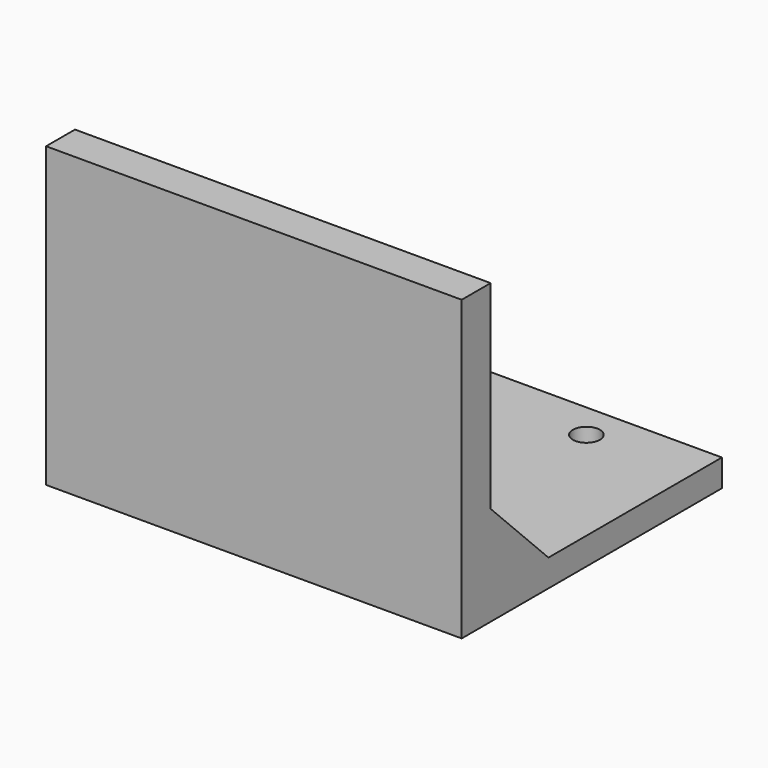
from build123d import *

# Parameters (mm, degrees)
F0_W      = 58.42
F0_H      = 45.72
F1_DEPTH  = 3.81
F2_W      = 58.42
F2_H      = 5.08
F3_DEPTH  = 38.1
F4_R      = 1.905
F5_DEPTH  = 3.811
F6_W      = 10.16
F6_H      = 10.16
F7_DEPTH  = 5.08
F8_SIZE   = 10.15999
F9_W      = 10.16
F9_H      = 10.16
F10_DEPTH = 5.08
F11_SIZE  = 10.15999


# Not quite as in the source:
# - a fillet or chamfer is up to 0.001 mm smaller than in the source, because OpenCascade refuses the exact size


with BuildPart() as f1:
    # F0 (on Top) → F1 (new body)
    with BuildSketch(Plane.XY):
        Rectangle(F0_W, F0_H)
    extrude(amount=F1_DEPTH)

    # F2 (on face) → F3 (join)
    with BuildSketch(Plane.XY.offset(3.81)):
        with Locations((0, -20.32)):
            Rectangle(F2_W, F2_H)
    extrude(amount=F3_DEPTH)

    # F4 (on face) → F5 (cut, through all)
    with BuildSketch(Plane.XY.offset(3.81)):
        with Locations((-14.224, 17.78)):
            Circle(F4_R)
        with Locations((14.224, 17.78)):
            Circle(F4_R)
        with Locations((14.224, -10.668)):
            Circle(F4_R)
        with Locations((-14.224, -10.668)):
            Circle(F4_R)
    extrude(amount=-F5_DEPTH, mode=Mode.SUBTRACT)

    # F6 (on face) → F7 (join)
    with BuildSketch(Plane(origin=(-29.21, 0, 0), x_dir=(0, -1, 0), z_dir=(-1, 0, 0))):
        with Locations((12.7, 8.89)):
            Rectangle(F6_W, F6_H)
    extrude(amount=-F7_DEPTH)

    # F8 (size 10.16 in the source; OpenCascade refuses exactly that, so slightly less here)
    f8_edges = [f1.edges().sort_by_distance(p)[0] for p in [
        (-26.67, -7.62, 13.97),
    ]]
    chamfer(f8_edges, length=F8_SIZE)

    # F9 (on face) → F10 (join)
    with BuildSketch(Plane.YZ.offset(29.21)):
        with Locations((-12.7, 8.89)):
            Rectangle(F9_W, F9_H)
    extrude(amount=-F10_DEPTH)

    # F11 (size 10.16 in the source; OpenCascade refuses exactly that, so slightly less here)
    f11_edges = [f1.edges().sort_by_distance(p)[0] for p in [
        (26.67, -7.62, 13.97),
    ]]
    chamfer(f11_edges, length=F11_SIZE)


solid = f1.part
